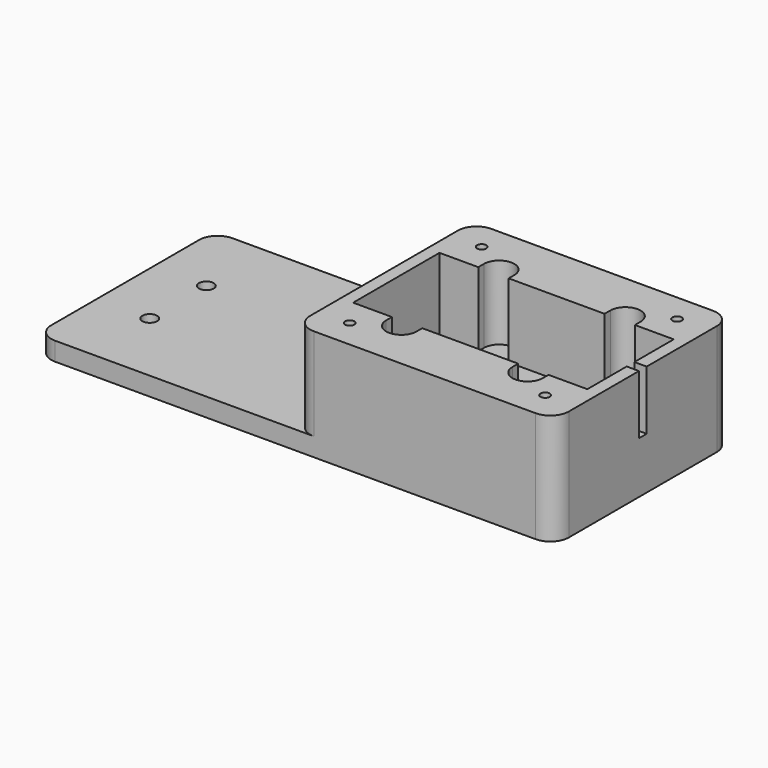
from build123d import *

# Parameters (mm, degrees)
F0_W          = 140
F0_H          = 60
F1_DEPTH      = 5
F2_W          = 70
F2_H          = 60
F3_DEPTH      = 25
F5_D          = 4
F6_R          = 5
F8_DEPTH      = 20
F10_D         = 2.5
F10_DEPTH     = 6
F10_TIP       = 0.7510757738
F11_W         = 3.325
F11_H         = 2.6
F12_DEPTH     = 16
F13_TEXT_SIZE = 20.8333333333
F14_DEPTH     = 1
F15_R         = 5


# Not quite as in the source:
# - Text() gives the source's letters only with a copy of the font that has no kerning and outlines rounded to 1/6400 em; it was checked with that copy


with BuildPart() as f1:
    # F0 (on Top) → F1 (new body)
    with BuildSketch(Plane.XY):
        Rectangle(F0_W, F0_H)
    extrude(amount=F1_DEPTH)

    # F2 (on face) → F3 (join)
    with BuildSketch(Plane.XY.offset(5)):
        with Locations((35, 0)):
            Rectangle(F2_W, F2_H)
    extrude(amount=F3_DEPTH)

    # F5 (through all)
    with Locations(Plane.XY.offset(5)):
        with Locations((-55.7, 9.56), (-55.7, -9.56)):
            Hole(F5_D / 2)

    # F6
    f6_edges = [f1.edges().sort_by_distance(p)[0] for p in [
        (-70, 30, 2.5),
        (-70, -30, 2.5),
    ]]
    fillet(f6_edges, radius=F6_R)

    # F7 (on face) → F8 (cut)
    with BuildSketch(Plane.XY.offset(30)):
        with BuildLine():
            Line((3.325, 14.6), (3.325, 0))
            Line((3.325, 0), (35, 0))
            Line((35, 0), (35, 14.6))
            Line((35, 14.6), (22.025, 14.6))
            Line((22.025, 14.6), (22.025, 16.528))
            ThreePointArc((22.025, 16.528), (17.925, 20.628), (13.825, 16.528))
            Line((13.825, 16.528), (13.825, 14.6))
            Line((13.825, 14.6), (3.325, 14.6))
        make_face()
        with BuildLine():
            Line((35, 0), (3.325, 0))
            Line((3.325, 0), (3.325, -14.6))
            Line((3.325, -14.6), (13.825, -14.6))
            Line((13.825, -14.6), (13.825, -16.528))
            ThreePointArc((13.825, -16.528), (17.925, -20.628), (22.025, -16.528))
            Line((22.025, -16.528), (22.025, -14.6))
            Line((22.025, -14.6), (35, -14.6))
            Line((35, -14.6), (35, 0))
        make_face()
        with BuildLine():
            Line((50.175, 0), (35, 0))
            Line((35, 0), (35, -14.6))
            Line((35, -14.6), (47.975, -14.6))
            Line((47.975, -14.6), (47.975, -16.528))
            ThreePointArc((47.975, -16.528), (52.075, -20.628), (56.175, -16.528))
            Line((56.175, -16.528), (56.175, -14.6))
            Line((56.175, -14.6), (66.675, -14.6))
            Line((66.675, -14.6), (66.675, -1.3))
            Line((66.675, -1.3), (66.675, 0))
            Line((66.675, 0), (61.175, 0))
            ThreePointArc((61.175, 0), (55.675, -5.5), (50.175, 0))
        make_face()
        with BuildLine():
            Line((35, 14.6), (35, 0))
            Line((35, 0), (50.175, 0))
            ThreePointArc((50.175, 0), (55.675, 5.5), (61.175, 0))
            Line((61.175, 0), (66.675, 0))
            Line((66.675, 0), (66.675, 1.3))
            Line((66.675, 1.3), (66.675, 14.6))
            Line((66.675, 14.6), (56.175, 14.6))
            Line((56.175, 14.6), (56.175, 16.528))
            ThreePointArc((56.175, 16.528), (52.075, 20.628), (47.975, 16.528))
            Line((47.975, 16.528), (47.975, 14.6))
            Line((47.975, 14.6), (35, 14.6))
        make_face()
        with BuildLine():
            Line((61.175, 0), (50.175, 0))
            ThreePointArc((50.175, 0), (55.675, -5.5), (61.175, 0))
        make_face()
        with BuildLine():
            ThreePointArc((61.175, 0), (55.675, 5.5), (50.175, 0))
            Line((50.175, 0), (61.175, 0))
        make_face()
    extrude(amount=-F8_DEPTH, mode=Mode.SUBTRACT)

    # F10
    with Locations(Plane.XY.offset(30)):
        with Locations((8.575, 22.3), (61.425, 22.3), (8.575, -22.3), (61.425, -22.3)):
            Hole(F10_D / 2, depth=F10_DEPTH)
            with Locations((0, 0, -(F10_DEPTH + F10_TIP / 2))):  # 118° drill point
                Cone(0, F10_D / 2, F10_TIP, mode=Mode.SUBTRACT)

    # F11 (on face) → F12 (cut)
    with BuildSketch(Plane.XY.offset(30)):
        with Locations((68.3375, 0)):
            Rectangle(F11_W, F11_H)
    extrude(amount=-F12_DEPTH, mode=Mode.SUBTRACT)

    # F13 (on face) → F14 (join)
    with BuildSketch(Plane(origin=(0, 0, 0), x_dir=(1, 0, 0), z_dir=(0, 0, -1))):
        with Locations((-38.3274739583, -7.5)):
            Text('EYE-CAS', F13_TEXT_SIZE, font='Open Sans', text_align=(TextAlign.LEFT, TextAlign.BOTTOM))
    extrude(amount=F14_DEPTH)

    # F15
    f15_edges = [f1.edges().sort_by_distance(p)[0] for p in [
        (0, -30, 17.5),
        (70, -30, 15),
        (70, 30, 15),
        (0, 30, 17.5),
    ]]
    fillet(f15_edges, radius=F15_R)


solid = f1.part
